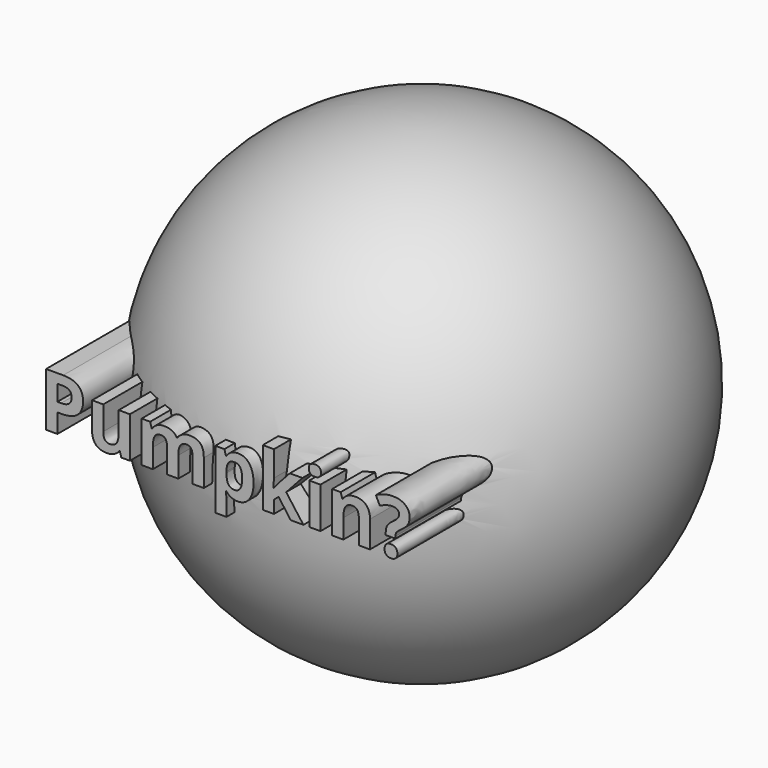
from build123d import *

# Parameters (mm, degrees)
F2_TEXT_SIZE = 20.3187300794
F3_DEPTH     = 66.04


# Not quite as in the source:
# - Text() gives the source's letters only with a copy of the font that has no kerning and outlines rounded to 1/6400 em; it was checked with that copy


with BuildPart() as f1:
    # F0 (on Front) → F1 (revolve)
    with BuildSketch(Plane.XZ):
        with BuildLine():
            Line((0, -63.5), (0, 63.5))
            ThreePointArc((0, 63.5), (-63.5, 0), (0, -63.5))
        make_face()
    revolve(axis=Axis((0, 0, 0), (0, 0, -1)))

    # F2 (on Front) → F3 (join)
    with BuildSketch(Plane.XZ):
        with Locations((-50.8, 0)):
            Text('Pumpkin?', F2_TEXT_SIZE, font='Open Sans', font_style=FontStyle.BOLD, text_align=(TextAlign.LEFT, TextAlign.BOTTOM))
    extrude(amount=F3_DEPTH)


solid = f1.part
